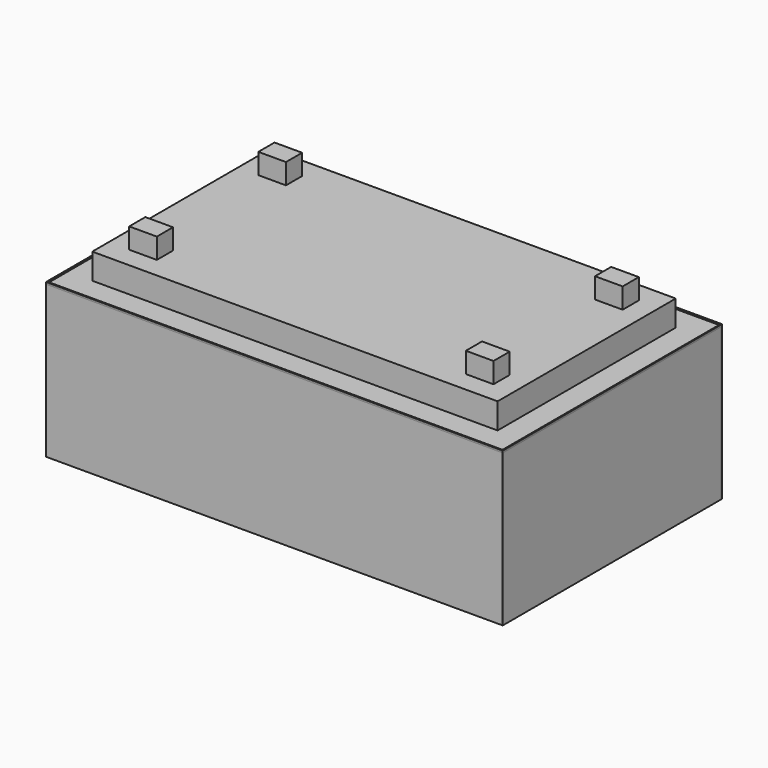
from build123d import *

# Parameters (mm, degrees)
F0_W      = 790
F0_H      = 434
F1_DEPTH  = 50
F2_W      = 890
F2_H      = 534
F3_DEPTH  = 2
F4_W      = 890
F4_H      = 2
F5_DEPTH  = 300
F6_W      = 890
F6_H      = 2
F7_DEPTH  = 300
F9_DEPTH  = 300
F10_W     = 886.24073763
F10_H     = 2
F11_DEPTH = 200
F14_W     = 53.8489925209
F14_H     = 39.3722521436
F15_DEPTH = 40


# Not quite as in the source:
# - the program builds the solid bodies; features that only make, move or delete a surface that nothing else refers to are left out


with BuildPart() as f1:
    # F0 (on Top) → F1 (new body)
    with BuildSketch(Plane.XY):
        Rectangle(F0_W, F0_H)
    extrude(amount=-F1_DEPTH)


with BuildPart() as f3:
    # F2 (on face) → F3 (new body)
    with BuildSketch(Plane(origin=(0, 0, -50), x_dir=(1, 0, 0), z_dir=(0, 0, -1))):
        Rectangle(F2_W, F2_H)
    extrude(amount=F3_DEPTH)


with BuildPart() as f5:
    # F4 (on face) → F5 (new body)
    with BuildSketch(Plane(origin=(0, 0, -52), x_dir=(1, 0, 0), z_dir=(0, 0, -1))):
        with Locations((0, 266)):
            Rectangle(F4_W, F4_H)
    extrude(amount=F5_DEPTH)


with BuildPart() as f7:
    # F6 (on face) → F7 (new body)
    with BuildSketch(Plane(origin=(0, 0, -52), x_dir=(1, 0, 0), z_dir=(0, 0, -1))):
        with Locations((0, -266)):
            Rectangle(F6_W, F6_H)
    extrude(amount=F7_DEPTH)


with BuildPart() as f9:
    # F8 (on face) → F9 (new body)
    with BuildSketch(Plane(origin=(0, 0, -52), x_dir=(1, 0, 0), z_dir=(0, 0, -1))):
        Polygon((-443, 264.9729303838), (-445, 264.9729303838), (-445, -265.0270696162), (-443.2746438212, -265.0279636871), align=None)
    extrude(amount=F9_DEPTH)


with BuildPart() as f9b:
    # F8 (on face) → F9, piece 2 (new body)
    with BuildSketch(Plane(origin=(0, 0, -52), x_dir=(1, 0, 0), z_dir=(0, 0, -1))):
        Polygon((445, -265.0270696162), (445, 264.9729303838), (443, 264.9729303838), (443.2746438214, -265.0279636871), align=None)
    extrude(amount=F9_DEPTH)


with BuildPart() as f11:
    # F10 (on face) → F11 (new body)
    with BuildSketch(Plane(origin=(0, 0, -52), x_dir=(1, 0, 0), z_dir=(0, 0, -1))):
        with Locations((0.1168335443, -124)):
            Rectangle(F10_W, F10_H)
    extrude(amount=F11_DEPTH)


with BuildPart() as f11_1:
    # F12: moved
    add(f11.part.moved(Location((0, 0, -96))))


with BuildPart() as f11_2:
    # F13: moved
    add(f11_1.part.moved(Location((0, 0, -4))))


with BuildPart() as f3_1:
    # F13: moved
    add(f3.part.moved(Location((0, 0, -4))))


with BuildPart() as f1_1:
    # F13: moved
    add(f1.part.moved(Location((0, 0, -4))))

    # F14 (on face) → F15 (join)
    with BuildSketch(Plane.XY.offset(-4)):
        with Locations((328.0755037396, 157.3138739282)):
            Rectangle(F14_W, F14_H)
        with Locations((-328.0755037396, -157.3138739282)):
            Rectangle(F14_W, F14_H)
        with Locations((328.0755037396, -157.3138739282)):
            Rectangle(F14_W, F14_H)
        with Locations((-328.0755037396, 157.3138739282)):
            Rectangle(F14_W, F14_H)
    extrude(amount=F15_DEPTH)


solid = Compound([f5.part, f7.part, f9.part, f9b.part, f11_2.part, f3_1.part, f1_1.part])
